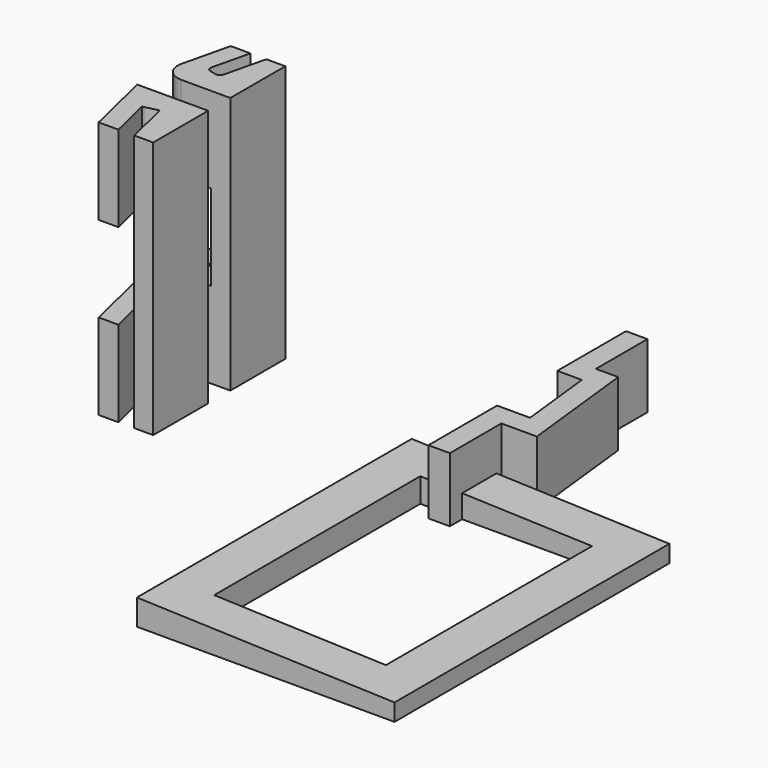
from build123d import *

# Parameters (mm, degrees)
F1_DEPTH  = 101.6
F2_W      = 50.8
F2_H      = 76.2
F3_DEPTH  = 7.621
F5_DEPTH  = 19.05
F7_DEPTH  = 76.2
F9_DEPTH  = 0.508
F10_DEPTH = 0.508
F12_DEPTH = 76.201
F8_W      = 15.24
F8_H      = 25.4
F13_DEPTH = 97.503062818
F15_R     = 5.08
F16_R     = 1.27


with BuildPart() as f1:
    # F0 (on Front) → F1 (new body)
    with BuildSketch(Plane.XZ):
        Polygon((0, 7.62), (0, 0), (76.2, 0), (76.2, 5.08), align=None)
    extrude(amount=F1_DEPTH)

    # F2 (on face) → F3 (cut, through all)
    with BuildSketch(Plane(origin=(0, 0, 0), x_dir=(1, 0, 0), z_dir=(0, 0, -1))):
        with Locations((38.1, 50.8)):
            Rectangle(F2_W, F2_H)
    extrude(amount=-F3_DEPTH, mode=Mode.SUBTRACT)


with BuildPart() as f5:
    # F4 (on Top) → F5 (new body)
    with BuildSketch(Plane.XY):
        Polygon((25.0658135089, 55.8246009568), (18.7158135089, 55.8246009568), (18.7158135089, 30.4246009568), (25.9808377175, 30.4246009568), (26.3358135089, 27.2496009568), (28.1138135089, 11.3466855008), (28.4687893003, 8.1716855008), (18.7158135089, 8.1716855008), (18.7158135089, -17.2283144992), (25.0658135089, -17.2283144992), (25.0658135089, 1.8216855008), (35.5683051289, 1.8216855008), (31.6604503803, 36.7746009568), (25.0658135089, 36.7746009568), align=None)
    extrude(amount=F5_DEPTH)


with BuildPart() as f7:
    # F6 (on Top) → F7 (new body)
    with BuildSketch(Plane.XY):
        Polygon((-62.001723196, -24.417937182), (-56.921723196, -24.417937182), (-56.921723196, -4.097937182), (-77.8925820998, -4.097937182), (-73.0516752635, -24.417937182), (-66.7016752635, -24.417937182), (-69.686772723, -11.8878095782), (-65.2392414078, -10.8282581634), align=None)
    extrude(amount=F7_DEPTH)

    # F9 (add): a face of the model
    f9_faces = [f7.faces().sort_by_distance(p)[0] for p in [
        (-63.6204823019, -17.6230976727, 38.1),
    ]]
    extrude(f9_faces, amount=F9_DEPTH)

    # F10 (cut): a face of the model
    f10_faces = [f7.faces().sort_by_distance(p)[0] for p in [
        (-68.1942239932, -18.1528733801, 38.1),
    ]]
    extrude(f10_faces, amount=-F10_DEPTH, mode=Mode.SUBTRACT)

    # F11 (on face) → F12 (cut, through all)
    with BuildSketch(Plane(origin=(0, 0, 0), x_dir=(1, 0, 0), z_dir=(0, 0, -1))):
        Polygon((-62.5239400924, 24.417937182), (-62.001723196, 24.417937182), (-62.4958933421, 24.5356651169), align=None)
        Polygon((-63.2905851658, 24.417937182), (-62.5239400924, 24.417937182), (-62.4958933421, 24.5356651169), align=None)
    extrude(amount=-F12_DEPTH, mode=Mode.SUBTRACT)

    # F8 (on face) → F13 (cut, through all)
    with BuildSketch(Plane(origin=(0, -4.097937182, 0), x_dir=(-1, 0, 0), z_dir=(0, 1, 0))):
        with Locations((70.2725820998, 38.1)):
            Rectangle(F8_W, F8_H)
    extrude(amount=-F13_DEPTH, mode=Mode.SUBTRACT)


with BuildPart() as f14_1:
    # F14: instance of F7
    add(f7.part.mirror(Plane.XZ))

    # F15
    f15_edges = [f14_1.edges().sort_by_distance(p)[0] for p in [
        (-77.892582, 4.097937, 12.7),
        (-77.892582, 4.097937, 63.5),
    ]]
    fillet(f15_edges, radius=F15_R)

    # F16
    f16_edges = [f14_1.edges().sort_by_distance(p)[0] for p in [
        (-65.733412, 10.945986, 63.5),
        (-65.733412, 10.945986, 12.7),
        (-70.180943, 12.005538, 12.7),
        (-70.180943, 12.005538, 63.5),
    ]]
    fillet(f16_edges, radius=F16_R)


solid = Compound([f1.part, f5.part, f7.part, f14_1.part])
